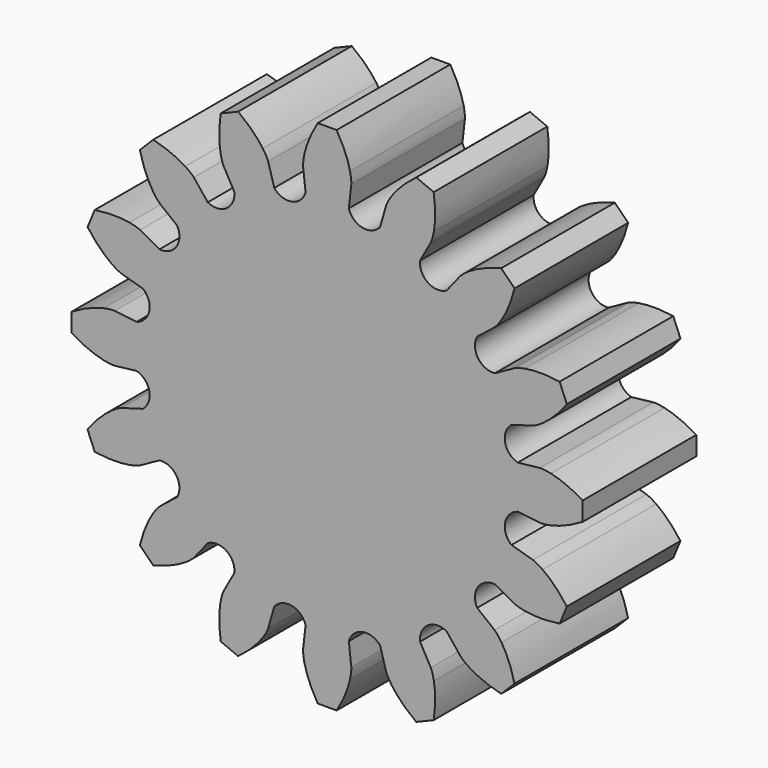
from build123d import *

# Parameters (mm, degrees)
F1_DEPTH = 6.35


# Not quite as in the source:
# - ends of sketch curves that miss each other by under 0.0002 mm in the source are joined


with BuildPart() as f1:
    # F0 (on Front) → F1 (new body)
    with BuildSketch(Plane.XZ):
        with BuildLine():
            ThreePointArc((8.2393478234, -2.3666267977), (7.9537993632, -1.582107911), (8.51783494, -0.9665823836))
            Line((8.51783494, -0.9665823836), (9.5076264, -1.0789158))
            add(Edge.make_bspline(
                [(9.5076264, -1.0789158), (9.562719, -1.0814812), (9.7264474, -1.0819638), (9.9996244, -1.022731)],
                knots=[0, 0, 0, 0, 1, 1, 1, 1], degree=3))
            add(Edge.make_bspline(
                [(9.9996244, -1.022731), (10.3372412, -0.9481566), (10.8256832, -0.7832852), (11.4238024, -0.4221988)],
                knots=[0, 0, 0, 0, 1, 1, 1, 1], degree=3))
            Line((11.4238024, -0.4221988), (11.4238024, 0.4221988))
            add(Edge.make_bspline(
                [(11.4238024, 0.4221988), (10.8256832, 0.7832852), (10.3372412, 0.9481566), (10.0005642, 1.0221722)],
                knots=[0, 0, 0, 0, 1, 1, 1, 1], degree=3))
            add(Edge.make_bspline(
                [(10.0005642, 1.0221722), (9.7264474, 1.0819638), (9.562719, 1.0814812), (9.5076264, 1.0789158)],
                knots=[0, 0, 0, 0, 1, 1, 1, 1], degree=3))
            Line((9.5076264, 1.0789158), (8.5178392, 0.966597))
            ThreePointArc((8.5178392, 0.966597), (7.9537993632, 1.582107911), (8.2393478234, 2.3666267977))
            Line((8.2393478234, 2.3666267977), (9.1967812, 2.6416254))
            add(Edge.make_bspline(
                [(9.1967812, 2.6416254), (9.2486734, 2.6603452), (9.4001082, 2.7225498), (9.6298258, 2.8818078)],
                knots=[0, 0, 0, 0, 1, 1, 1, 1], degree=3))
            add(Edge.make_bspline(
                [(9.6298258, 2.8818078), (9.9132136, 3.0799024), (10.3013764, 3.4191448), (10.7157774, 3.9816532)],
                knots=[0, 0, 0, 0, 1, 1, 1, 1], degree=3))
            Line((10.7157774, 3.9816532), (10.392664, 4.7617634))
            add(Edge.make_bspline(
                [(10.392664, 4.7617634), (9.7018856, 4.8664622), (9.1875102, 4.8318674), (8.8481408, 4.7714154)],
                knots=[0, 0, 0, 0, 1, 1, 1, 1], degree=3))
            add(Edge.make_bspline(
                [(8.8481408, 4.7714154), (8.5720174, 4.721733), (8.4209382, 4.6586394), (8.3710272, 4.6351952)],
                knots=[0, 0, 0, 0, 1, 1, 1, 1], degree=3))
            Line((8.3710272, 4.6351952), (7.4995532, 4.152646))
            ThreePointArc((7.4995532, 4.152646), (6.74291272, 4.5054747374), (6.7064897747, 5.339536775))
            Line((6.7064897747, 5.339536775), (7.4858118, 5.9600084))
            add(Edge.make_bspline(
                [(7.4858118, 5.9600084), (7.5265788, 5.9971432), (7.6426822, 6.1125862), (7.7939646, 6.3476124)],
                knots=[0, 0, 0, 0, 1, 1, 1, 1], degree=3))
            add(Edge.make_bspline(
                [(7.7939646, 6.3476124), (7.9799688, 6.6390774), (8.208772, 7.1010526), (8.3763866, 7.7793088)],
                knots=[0, 0, 0, 0, 1, 1, 1, 1], degree=3))
            Line((8.3763866, 7.7793088), (7.7793088, 8.3763866))
            add(Edge.make_bspline(
                [(7.7793088, 8.3763866), (7.1010526, 8.208772), (6.6390774, 7.9799688), (6.3486792, 7.794244)],
                knots=[0, 0, 0, 0, 1, 1, 1, 1], degree=3))
            add(Edge.make_bspline(
                [(6.3486792, 7.794244), (6.1125862, 7.6426822), (5.9971432, 7.5265788), (5.9600084, 7.4858118)],
                knots=[0, 0, 0, 0, 1, 1, 1, 1], degree=3))
            Line((5.9600084, 7.4858118), (5.3395372, 6.706489))
            ThreePointArc((5.3395372, 6.706489), (4.5054747374, 6.74291272), (4.1526538272, 7.4995523427))
            Line((4.1526538272, 7.4995523427), (4.6351952, 8.3710272))
            add(Edge.make_bspline(
                [(4.6351952, 8.3710272), (4.6586394, 8.4209382), (4.721733, 8.5720174), (4.7715678, 8.847074)],
                knots=[0, 0, 0, 0, 1, 1, 1, 1], degree=3))
            add(Edge.make_bspline(
                [(4.7715678, 8.847074), (4.8318674, 9.1875102), (4.8664622, 9.7018856), (4.7617634, 10.392664)],
                knots=[0, 0, 0, 0, 1, 1, 1, 1], degree=3))
            Line((4.7617634, 10.392664), (3.9816532, 10.7157774))
            add(Edge.make_bspline(
                [(3.9816532, 10.7157774), (3.4191448, 10.3013764), (3.0799024, 9.9132136), (2.8826968, 9.6304862)],
                knots=[0, 0, 0, 0, 1, 1, 1, 1], degree=3))
            add(Edge.make_bspline(
                [(2.8826968, 9.6304862), (2.7225498, 9.4001082), (2.6603452, 9.2486734), (2.6416254, 9.1967812)],
                knots=[0, 0, 0, 0, 1, 1, 1, 1], degree=3))
            Line((2.6416254, 9.1967812), (2.3666196, 8.2393536))
            ThreePointArc((2.3666196, 8.2393536), (1.582107911, 7.9537993632), (0.9665823836, 8.51783494))
            Line((0.9665823836, 8.51783494), (1.0789158, 9.5076264))
            add(Edge.make_bspline(
                [(1.0789158, 9.5076264), (1.0814812, 9.562719), (1.0819638, 9.7264474), (1.022731, 9.9996244)],
                knots=[0, 0, 0, 0, 1, 1, 1, 1], degree=3))
            add(Edge.make_bspline(
                [(1.022731, 9.9996244), (0.9481566, 10.3372412), (0.7832852, 10.8256832), (0.4221988, 11.4238024)],
                knots=[0, 0, 0, 0, 1, 1, 1, 1], degree=3))
            Line((0.4221988, 11.4238024), (-0.4221988, 11.4238024))
            add(Edge.make_bspline(
                [(-0.4221988, 11.4238024), (-0.7832852, 10.8256832), (-0.9481566, 10.3372412), (-1.0221722, 10.0005642)],
                knots=[0, 0, 0, 0, 1, 1, 1, 1], degree=3))
            add(Edge.make_bspline(
                [(-1.0221722, 10.0005642), (-1.0819638, 9.7264474), (-1.0814812, 9.562719), (-1.0789158, 9.5076264)],
                knots=[0, 0, 0, 0, 1, 1, 1, 1], degree=3))
            Line((-1.0789158, 9.5076264), (-0.966597, 8.5178392))
            ThreePointArc((-0.966597, 8.5178392), (-1.582107911, 7.9537993632), (-2.3666267977, 8.2393478234))
            Line((-2.3666267977, 8.2393478234), (-2.6416254, 9.1967812))
            add(Edge.make_bspline(
                [(-2.6416254, 9.1967812), (-2.6603452, 9.2486734), (-2.7225498, 9.4001082), (-2.8818078, 9.6298258)],
                knots=[0, 0, 0, 0, 1, 1, 1, 1], degree=3))
            add(Edge.make_bspline(
                [(-2.8818078, 9.6298258), (-3.0799024, 9.9132136), (-3.4191448, 10.3013764), (-3.9816532, 10.7157774)],
                knots=[0, 0, 0, 0, 1, 1, 1, 1], degree=3))
            Line((-3.9816532, 10.7157774), (-4.7617634, 10.392664))
            add(Edge.make_bspline(
                [(-4.7617634, 10.392664), (-4.8664622, 9.7018856), (-4.8318674, 9.1875102), (-4.7714154, 8.8481408)],
                knots=[0, 0, 0, 0, 1, 1, 1, 1], degree=3))
            add(Edge.make_bspline(
                [(-4.7714154, 8.8481408), (-4.721733, 8.5720174), (-4.6586394, 8.4209382), (-4.6351952, 8.3710272)],
                knots=[0, 0, 0, 0, 1, 1, 1, 1], degree=3))
            Line((-4.6351952, 8.3710272), (-4.152646, 7.4995532))
            ThreePointArc((-4.152646, 7.4995532), (-4.5054747374, 6.74291272), (-5.339536775, 6.7064897747))
            Line((-5.339536775, 6.7064897747), (-5.9600084, 7.4858118))
            add(Edge.make_bspline(
                [(-5.9600084, 7.4858118), (-5.9971432, 7.5265788), (-6.1125862, 7.6426822), (-6.3476124, 7.7939646)],
                knots=[0, 0, 0, 0, 1, 1, 1, 1], degree=3))
            add(Edge.make_bspline(
                [(-6.3476124, 7.7939646), (-6.6390774, 7.9799688), (-7.1010526, 8.208772), (-7.7793088, 8.3763866)],
                knots=[0, 0, 0, 0, 1, 1, 1, 1], degree=3))
            Line((-7.7793088, 8.3763866), (-8.3763866, 7.7793088))
            add(Edge.make_bspline(
                [(-8.3763866, 7.7793088), (-8.208772, 7.1010526), (-7.9799688, 6.6390774), (-7.794244, 6.3486792)],
                knots=[0, 0, 0, 0, 1, 1, 1, 1], degree=3))
            add(Edge.make_bspline(
                [(-7.794244, 6.3486792), (-7.6426822, 6.1125862), (-7.5265788, 5.9971432), (-7.4858118, 5.9600084)],
                knots=[0, 0, 0, 0, 1, 1, 1, 1], degree=3))
            Line((-7.4858118, 5.9600084), (-6.706489, 5.3395372))
            ThreePointArc((-6.706489, 5.3395372), (-6.74291272, 4.5054747374), (-7.4995523427, 4.1526538272))
            Line((-7.4995523427, 4.1526538272), (-8.3710272, 4.6351952))
            add(Edge.make_bspline(
                [(-8.3710272, 4.6351952), (-8.4209382, 4.6586394), (-8.5720174, 4.721733), (-8.847074, 4.7715678)],
                knots=[0, 0, 0, 0, 1, 1, 1, 1], degree=3))
            add(Edge.make_bspline(
                [(-8.847074, 4.7715678), (-9.1875102, 4.8318674), (-9.7018856, 4.8664622), (-10.392664, 4.7617634)],
                knots=[0, 0, 0, 0, 1, 1, 1, 1], degree=3))
            Line((-10.392664, 4.7617634), (-10.7157774, 3.9816532))
            add(Edge.make_bspline(
                [(-10.7157774, 3.9816532), (-10.3013764, 3.4191448), (-9.9132136, 3.0799024), (-9.6304862, 2.8826968)],
                knots=[0, 0, 0, 0, 1, 1, 1, 1], degree=3))
            add(Edge.make_bspline(
                [(-9.6304862, 2.8826968), (-9.4001082, 2.7225498), (-9.2486734, 2.6603452), (-9.1967812, 2.6416254)],
                knots=[0, 0, 0, 0, 1, 1, 1, 1], degree=3))
            Line((-9.1967812, 2.6416254), (-8.2393536, 2.3666196))
            ThreePointArc((-8.2393536, 2.3666196), (-7.9537993632, 1.582107911), (-8.51783494, 0.9665823836))
            Line((-8.51783494, 0.9665823836), (-9.5076264, 1.0789158))
            add(Edge.make_bspline(
                [(-9.5076264, 1.0789158), (-9.562719, 1.0814812), (-9.7264474, 1.0819638), (-9.9996244, 1.022731)],
                knots=[0, 0, 0, 0, 1, 1, 1, 1], degree=3))
            add(Edge.make_bspline(
                [(-9.9996244, 1.022731), (-10.3372412, 0.9481566), (-10.8256832, 0.7832852), (-11.4238024, 0.4221988)],
                knots=[0, 0, 0, 0, 1, 1, 1, 1], degree=3))
            Line((-11.4238024, 0.4221988), (-11.4238024, -0.4221988))
            add(Edge.make_bspline(
                [(-11.4238024, -0.4221988), (-10.8256832, -0.7832852), (-10.3372412, -0.9481566), (-10.0005642, -1.0221722)],
                knots=[0, 0, 0, 0, 1, 1, 1, 1], degree=3))
            add(Edge.make_bspline(
                [(-10.0005642, -1.0221722), (-9.7264474, -1.0819638), (-9.562719, -1.0814812), (-9.5076264, -1.0789158)],
                knots=[0, 0, 0, 0, 1, 1, 1, 1], degree=3))
            Line((-9.5076264, -1.0789158), (-8.5178392, -0.966597))
            ThreePointArc((-8.5178392, -0.966597), (-7.9537993632, -1.582107911), (-8.2393478234, -2.3666267977))
            Line((-8.2393478234, -2.3666267977), (-9.1967812, -2.6416254))
            add(Edge.make_bspline(
                [(-9.1967812, -2.6416254), (-9.2486734, -2.6603452), (-9.4001082, -2.7225498), (-9.6298258, -2.8818078)],
                knots=[0, 0, 0, 0, 1, 1, 1, 1], degree=3))
            add(Edge.make_bspline(
                [(-9.6298258, -2.8818078), (-9.9132136, -3.0799024), (-10.3013764, -3.4191448), (-10.7157774, -3.9816532)],
                knots=[0, 0, 0, 0, 1, 1, 1, 1], degree=3))
            Line((-10.7157774, -3.9816532), (-10.392664, -4.7617634))
            add(Edge.make_bspline(
                [(-10.392664, -4.7617634), (-9.7018856, -4.8664622), (-9.1875102, -4.8318674), (-8.8481408, -4.7714154)],
                knots=[0, 0, 0, 0, 1, 1, 1, 1], degree=3))
            add(Edge.make_bspline(
                [(-8.8481408, -4.7714154), (-8.5720174, -4.721733), (-8.4209382, -4.6586394), (-8.3710272, -4.6351952)],
                knots=[0, 0, 0, 0, 1, 1, 1, 1], degree=3))
            Line((-8.3710272, -4.6351952), (-7.4995532, -4.152646))
            ThreePointArc((-7.4995532, -4.152646), (-6.74291272, -4.5054747374), (-6.7064897747, -5.339536775))
            Line((-6.7064897747, -5.339536775), (-7.4858118, -5.9600084))
            add(Edge.make_bspline(
                [(-7.4858118, -5.9600084), (-7.5265788, -5.9971432), (-7.6426822, -6.1125862), (-7.7939646, -6.3476124)],
                knots=[0, 0, 0, 0, 1, 1, 1, 1], degree=3))
            add(Edge.make_bspline(
                [(-7.7939646, -6.3476124), (-7.9799688, -6.6390774), (-8.208772, -7.1010526), (-8.3763866, -7.7793088)],
                knots=[0, 0, 0, 0, 1, 1, 1, 1], degree=3))
            Line((-8.3763866, -7.7793088), (-7.7793088, -8.3763866))
            add(Edge.make_bspline(
                [(-7.7793088, -8.3763866), (-7.1010526, -8.208772), (-6.6390774, -7.9799688), (-6.3486792, -7.794244)],
                knots=[0, 0, 0, 0, 1, 1, 1, 1], degree=3))
            add(Edge.make_bspline(
                [(-6.3486792, -7.794244), (-6.1125862, -7.6426822), (-5.9971432, -7.5265788), (-5.9600084, -7.4858118)],
                knots=[0, 0, 0, 0, 1, 1, 1, 1], degree=3))
            Line((-5.9600084, -7.4858118), (-5.3395372, -6.706489))
            ThreePointArc((-5.3395372, -6.706489), (-4.5054747374, -6.74291272), (-4.1526538272, -7.4995523427))
            Line((-4.1526538272, -7.4995523427), (-4.6351952, -8.3710272))
            add(Edge.make_bspline(
                [(-4.6351952, -8.3710272), (-4.6586394, -8.4209382), (-4.721733, -8.5720174), (-4.7715678, -8.847074)],
                knots=[0, 0, 0, 0, 1, 1, 1, 1], degree=3))
            add(Edge.make_bspline(
                [(-4.7715678, -8.847074), (-4.8318674, -9.1875102), (-4.8664622, -9.7018856), (-4.7617634, -10.392664)],
                knots=[0, 0, 0, 0, 1, 1, 1, 1], degree=3))
            Line((-4.7617634, -10.392664), (-3.9816532, -10.7157774))
            add(Edge.make_bspline(
                [(-3.9816532, -10.7157774), (-3.4191448, -10.3013764), (-3.0799024, -9.9132136), (-2.8826968, -9.6304862)],
                knots=[0, 0, 0, 0, 1, 1, 1, 1], degree=3))
            add(Edge.make_bspline(
                [(-2.8826968, -9.6304862), (-2.7225498, -9.4001082), (-2.6603452, -9.2486734), (-2.6416254, -9.1967812)],
                knots=[0, 0, 0, 0, 1, 1, 1, 1], degree=3))
            Line((-2.6416254, -9.1967812), (-2.3666196, -8.2393536))
            ThreePointArc((-2.3666196, -8.2393536), (-1.582107911, -7.9537993632), (-0.9665823836, -8.51783494))
            Line((-0.9665823836, -8.51783494), (-1.0789158, -9.5076264))
            add(Edge.make_bspline(
                [(-1.0789158, -9.5076264), (-1.0814812, -9.562719), (-1.0819638, -9.7264474), (-1.022731, -9.9996244)],
                knots=[0, 0, 0, 0, 1, 1, 1, 1], degree=3))
            add(Edge.make_bspline(
                [(-1.022731, -9.9996244), (-0.9481566, -10.3372412), (-0.7832852, -10.8256832), (-0.4221988, -11.4238024)],
                knots=[0, 0, 0, 0, 1, 1, 1, 1], degree=3))
            Line((-0.4221988, -11.4238024), (0.4221988, -11.4238024))
            add(Edge.make_bspline(
                [(0.4221988, -11.4238024), (0.7832852, -10.8256832), (0.9481566, -10.3372412), (1.0221722, -10.0005642)],
                knots=[0, 0, 0, 0, 1, 1, 1, 1], degree=3))
            add(Edge.make_bspline(
                [(1.0221722, -10.0005642), (1.0819638, -9.7264474), (1.0814812, -9.562719), (1.0789158, -9.5076264)],
                knots=[0, 0, 0, 0, 1, 1, 1, 1], degree=3))
            Line((1.0789158, -9.5076264), (0.966597, -8.5178392))
            ThreePointArc((0.966597, -8.5178392), (1.582107911, -7.9537993632), (2.3666267977, -8.2393478234))
            Line((2.3666267977, -8.2393478234), (2.6416254, -9.1967812))
            add(Edge.make_bspline(
                [(2.6416254, -9.1967812), (2.6603452, -9.2486734), (2.7225498, -9.4001082), (2.8818078, -9.6298258)],
                knots=[0, 0, 0, 0, 1, 1, 1, 1], degree=3))
            add(Edge.make_bspline(
                [(2.8818078, -9.6298258), (3.0799024, -9.9132136), (3.4191448, -10.3013764), (3.9816532, -10.7157774)],
                knots=[0, 0, 0, 0, 1, 1, 1, 1], degree=3))
            Line((3.9816532, -10.7157774), (4.7617634, -10.392664))
            add(Edge.make_bspline(
                [(4.7617634, -10.392664), (4.8664622, -9.7018856), (4.8318674, -9.1875102), (4.7714154, -8.8481408)],
                knots=[0, 0, 0, 0, 1, 1, 1, 1], degree=3))
            add(Edge.make_bspline(
                [(4.7714154, -8.8481408), (4.721733, -8.5720174), (4.6586394, -8.4209382), (4.6351952, -8.3710272)],
                knots=[0, 0, 0, 0, 1, 1, 1, 1], degree=3))
            Line((4.6351952, -8.3710272), (4.152646, -7.4995532))
            ThreePointArc((4.152646, -7.4995532), (4.5054747374, -6.74291272), (5.339536775, -6.7064897747))
            Line((5.339536775, -6.7064897747), (5.9600084, -7.4858118))
            add(Edge.make_bspline(
                [(5.9600084, -7.4858118), (5.9971432, -7.5265788), (6.1125862, -7.6426822), (6.3476124, -7.7939646)],
                knots=[0, 0, 0, 0, 1, 1, 1, 1], degree=3))
            add(Edge.make_bspline(
                [(6.3476124, -7.7939646), (6.6390774, -7.9799688), (7.1010526, -8.208772), (7.7793088, -8.3763866)],
                knots=[0, 0, 0, 0, 1, 1, 1, 1], degree=3))
            Line((7.7793088, -8.3763866), (8.3763866, -7.7793088))
            add(Edge.make_bspline(
                [(8.3763866, -7.7793088), (8.208772, -7.1010526), (7.9799688, -6.6390774), (7.794244, -6.3486792)],
                knots=[0, 0, 0, 0, 1, 1, 1, 1], degree=3))
            add(Edge.make_bspline(
                [(7.794244, -6.3486792), (7.6426822, -6.1125862), (7.5265788, -5.9971432), (7.4858118, -5.9600084)],
                knots=[0, 0, 0, 0, 1, 1, 1, 1], degree=3))
            Line((7.4858118, -5.9600084), (6.706489, -5.3395372))
            ThreePointArc((6.706489, -5.3395372), (6.74291272, -4.5054747374), (7.4995523427, -4.1526538272))
            Line((7.4995523427, -4.1526538272), (8.3710272, -4.6351952))
            add(Edge.make_bspline(
                [(8.3710272, -4.6351952), (8.4209382, -4.6586394), (8.5720174, -4.721733), (8.847074, -4.7715678)],
                knots=[0, 0, 0, 0, 1, 1, 1, 1], degree=3))
            add(Edge.make_bspline(
                [(8.847074, -4.7715678), (9.1875102, -4.8318674), (9.7018856, -4.8664622), (10.392664, -4.7617634)],
                knots=[0, 0, 0, 0, 1, 1, 1, 1], degree=3))
            Line((10.392664, -4.7617634), (10.7157774, -3.9816532))
            add(Edge.make_bspline(
                [(10.7157774, -3.9816532), (10.3013764, -3.4191448), (9.9132136, -3.0799024), (9.6304862, -2.8826968)],
                knots=[0, 0, 0, 0, 1, 1, 1, 1], degree=3))
            add(Edge.make_bspline(
                [(9.6304862, -2.8826968), (9.4001082, -2.7225498), (9.2486734, -2.6603452), (9.1967812, -2.6416254)],
                knots=[0, 0, 0, 0, 1, 1, 1, 1], degree=3))
            Line((9.1967812, -2.6416254), (8.2393478234, -2.3666267977))
        make_face()
    extrude(amount=F1_DEPTH)


solid = f1.part
